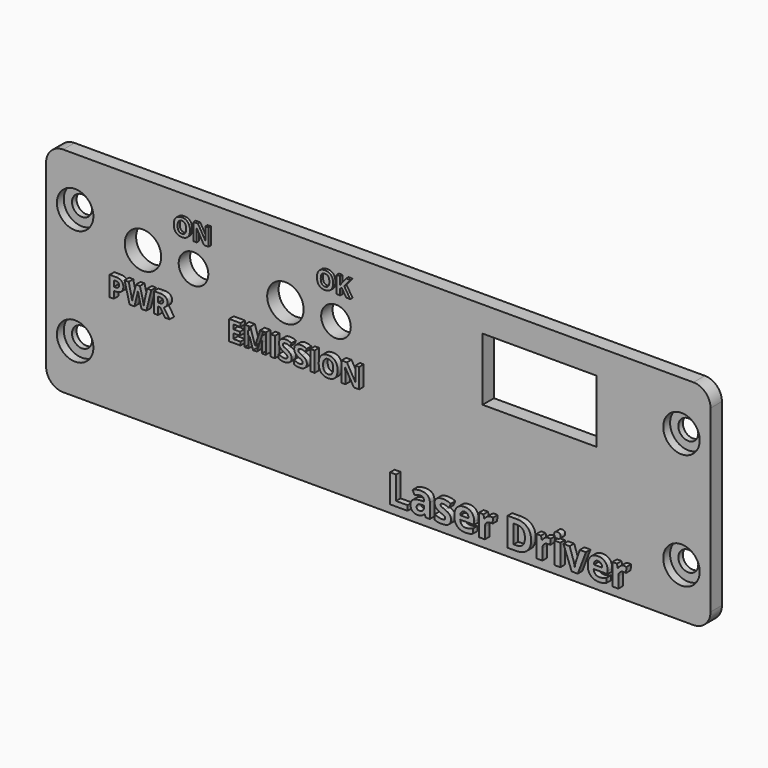
from build123d import *

# Parameters (mm, degrees)
F0_R          = 1.75
F1_DEPTH      = 2.5
F2_R          = 3.2
F3_DEPTH      = 1.5
F4_W          = 2.5
F4_H          = 6
F5_DEPTH      = 1.25
F6_R          = 3.2
F6_R_2        = 2.6
F7_DEPTH      = 2.501
F9_DEPTH      = 2.501
F10_TEXT_SIZE = 4.8611111111
F11_DEPTH     = 1
F12_TEXT_SIZE = 6.9444444444
F13_DEPTH     = 1
F14_TEXT_SIZE = 4.1666666667
F15_DEPTH     = 0.5


# Not quite as in the source:
# - a feature names something its author has since deleted; it is built from what else it names
# - Text() gives the source's letters only with a copy of the font that has no kerning and outlines rounded to 1/6400 em; it was checked with that copy


with BuildPart() as f1:
    # F0 (on Front) → F1 (new body)
    with BuildSketch(Plane.XZ):
        with BuildLine():
            Line((55.3, 18.75), (-55.3, 18.75))
            ThreePointArc((-55.3, 18.75), (-57.4213203436, 17.8713203436), (-58.3, 15.75))
            Line((-58.3, 15.75), (-58.3, -15.75))
            ThreePointArc((-58.3, -15.75), (-57.4213203436, -17.8713203436), (-55.3, -18.75))
            Line((-55.3, -18.75), (55.3, -18.75))
            ThreePointArc((55.3, -18.75), (57.4213203436, -17.8713203436), (58.3, -15.75))
            Line((58.3, -15.75), (58.3, 15.75))
            ThreePointArc((58.3, 15.75), (57.4213203436, 17.8713203436), (55.3, 18.75))
        make_face()
        with Locations((-53.2, -10.15)):
            Circle(F0_R, mode=Mode.SUBTRACT)
        with Locations((53.2, -10.15)):
            Circle(F0_R, mode=Mode.SUBTRACT)
        with Locations((-53.2, 10.15)):
            Circle(F0_R, mode=Mode.SUBTRACT)
        with Locations((53.2, 10.15)):
            Circle(F0_R, mode=Mode.SUBTRACT)
    extrude(amount=F1_DEPTH)

    # F2 (on face) → F3 (cut)
    with BuildSketch(Plane.XZ.offset(2.5)):
        with Locations((-53.2, 10.15)):
            Circle(F2_R)
        with Locations((53.2, 10.15)):
            Circle(F2_R)
        with Locations((-53.2, -10.15)):
            Circle(F2_R)
        with Locations((53.2, -10.15)):
            Circle(F2_R)
    extrude(amount=-F3_DEPTH, mode=Mode.SUBTRACT)

    # F4 (on face) → F5 (cut)
    with BuildSketch(Plane(origin=(0, 0, 0), x_dir=(-1, 0, 0), z_dir=(0, 1, 0))):
        with Locations((57.05, 0)):
            Rectangle(F4_W, F4_H)
    extrude(amount=-F5_DEPTH, mode=Mode.SUBTRACT)

    # F6 (on face) → F7 (cut, through all)
    with BuildSketch(Plane.XZ.offset(2.5)):
        with Locations((-41.3, 7.75)):
            Circle(F6_R)
        with Locations((-32.4288010597, 7.75)):
            Circle(F6_R_2)
        with Locations((-16.3, 7.75)):
            Circle(F6_R)
        with Locations((-7.4288010597, 7.75)):
            Circle(F6_R_2)
    extrude(amount=-F7_DEPTH, mode=Mode.SUBTRACT)

    # F8 (on face) → F9 (cut, through all)
    with BuildSketch(Plane.XZ.offset(2.5)):
        Polygon((38.3, 14.25), (28.3, 14.25), (18.3, 14.25), (18.3, 3.25), (28.3, 3.25), (38.3, 3.25), align=None)
    extrude(amount=-F9_DEPTH, mode=Mode.SUBTRACT)

    # F10 (on face) → F11 (join)
    with BuildSketch(Plane.XZ.offset(2.5)):
        with Locations((-46.7809027778, -0.75)):
            Text('PWR', F10_TEXT_SIZE, font='Open Sans', font_style=FontStyle.BOLD, text_align=(TextAlign.LEFT, TextAlign.BOTTOM))
        with Locations((-25.8190972222, -0.75)):
            Text('EMISSION', F10_TEXT_SIZE, font='Open Sans', font_style=FontStyle.BOLD, text_align=(TextAlign.LEFT, TextAlign.BOTTOM))
    extrude(amount=F11_DEPTH)

    # F12 (on face) → F13 (join)
    with BuildSketch(Plane.XZ.offset(2.5)):
        with Locations((2.2474826389, -16.75)):
            Text('Laser Driver', F12_TEXT_SIZE, font='Open Sans', font_style=FontStyle.BOLD, text_align=(TextAlign.LEFT, TextAlign.BOTTOM))
    extrude(amount=F13_DEPTH)

    # F14 (on face) → F15 (join)
    with BuildSketch(Plane.XZ.offset(2.5)):
        with Locations((-35.7286057472, 12.35)):
            Text('ON', F14_TEXT_SIZE, font='Open Sans', font_style=FontStyle.BOLD, text_align=(TextAlign.LEFT, TextAlign.BOTTOM))
        with Locations((-10.6055588722, 12.35)):
            Text('OK', F14_TEXT_SIZE, font='Open Sans', font_style=FontStyle.BOLD, text_align=(TextAlign.LEFT, TextAlign.BOTTOM))
    extrude(amount=F15_DEPTH)


solid = f1.part
